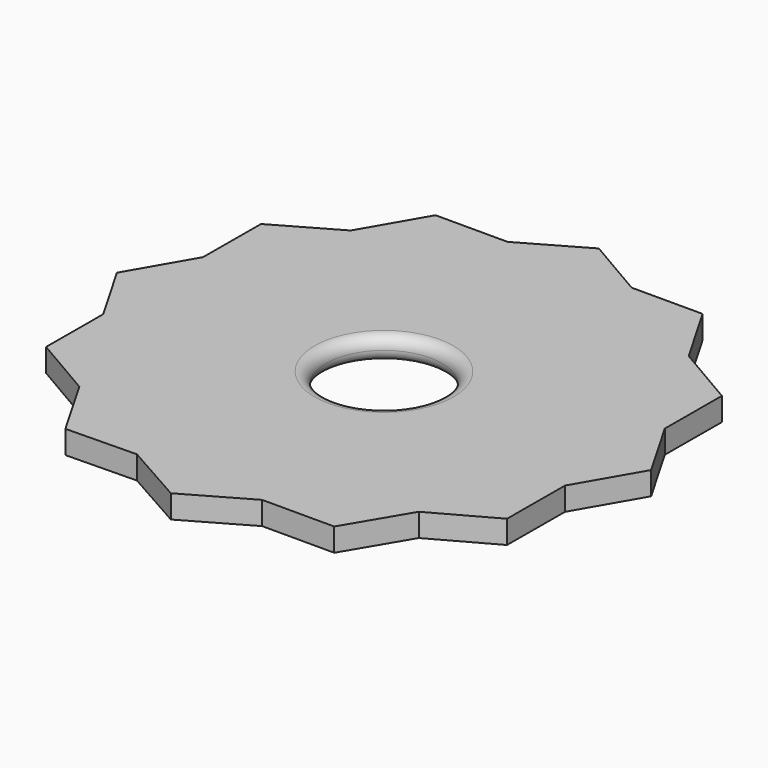
from build123d import *

# Parameters (mm, degrees)
F0_R     = 6.35
F1_DEPTH = 2.54
F2_R     = 1.26999


# Not quite as in the source:
# - a fillet or chamfer is up to 0.001 mm smaller than in the source, because OpenCascade refuses the exact size


with BuildPart() as f1:
    # F0 (on Top) → F1 (new body)
    with BuildSketch(Plane.XY):
        with BuildLine():
            Line((0.1342973504, 29.3290862039), (12.5991438484, 22.0549671115))
            ThreePointArc((12.5991438484, 22.0549671115), (12.7000000903, 21.997045204), (12.8005900541, 21.9386620893))
            Line((12.8005900541, 21.9386620893), (6.8682756911, 25.4))
            Line((6.8682756911, 25.4), (0.1342973504, 29.3290862039))
        make_face()
        with BuildLine():
            ThreePointArc((-12.5991438484, 22.0549671115), (0, 25.4), (12.5991438484, 22.0549671115))
            Line((12.5991438484, 22.0549671115), (0.1342973504, 29.3290862039))
            Line((0.1342973504, 29.3290862039), (-6.7436197563, 25.4))
            Line((-6.7436197563, 25.4), (-12.5991438484, 22.0549671115))
        make_face()
        Polygon((-18.5629074106, 18.6481012287), (-12.5991438484, 22.0549671115), (-6.7436197563, 25.4), (-14.6646968374, 25.4), align=None)
        with BuildLine():
            ThreePointArc((-25.3997337218, 0.1163050384), (-21.9386621638, 12.8005899263), (-12.5991438484, 22.0549671115))
            Line((-12.5991438484, 22.0549671115), (-18.5629074106, 18.6481012287))
            Line((-18.5629074106, 18.6481012287), (-25.3325850472, 14.780848019))
            Line((-25.3325850472, 14.780848019), (-25.3688551343, 6.8598539776))
            Line((-25.3688551343, 6.8598539776), (-25.3997337218, 0.1163050384))
        make_face()
        with BuildLine():
            Line((18.625235378, 18.5401460224), (12.8005900541, 21.9386620893))
            ThreePointArc((12.8005900541, 21.9386620893), (12.8993470878, 21.8807414113), (12.9978420445, 21.822376181))
            Line((12.9978420446, 21.822376181), (25.4668823975, 14.5482381848))
            Line((25.4668823975, 14.5482381848), (18.625235378, 18.5401460224))
        make_face()
        Polygon((6.8682756911, 25.4), (12.8005900541, 21.9386620893), (18.625235378, 18.5401460224), (14.6646968374, 25.4), align=None)
        with BuildLine():
            Line((25.4668823975, 14.5482381848), (12.9978420446, 21.822376181))
            ThreePointArc((12.9978420445, 21.822376181), (22.0828574683, 12.550195458), (25.4, 0))
            ThreePointArc((25.4, 0), (25.3999334305, -0.0581525957), (25.3997337225, -0.1163048866))
            Line((25.3997337225, -0.1163048866), (25.4002662804, 0))
            Line((25.4002662804, 0), (25.4311831017, 6.7518987713))
            Line((25.4311831017, 6.7518987713), (25.4668823975, 14.5482381848))
        make_face()
        Polygon((-25.4002662804, 0), (-25.3997337218, 0.1163050384), (-25.3688551343, 6.8598539776), (-29.3293936748, 0), (-25.4311831017, -6.7518987713), align=None)
        with BuildLine():
            ThreePointArc((-21.9970455091, -12.6999995618), (-24.5495027703, -6.5178151043), (-25.3997337218, 0.1163050384))
            Line((-25.3997337218, 0.1163050384), (-25.4002662804, 0))
            Line((-25.4002662804, 0), (-25.4311831017, -6.7518987713))
            Line((-25.4311831017, -6.7518987713), (-21.9970455091, -12.6999995618))
        make_face()
        with BuildLine():
            ThreePointArc((-12.800589874, -21.9386621944), (-18.0015854544, -17.9193448856), (-21.9970455091, -12.6999995618))
            Line((-21.9970455091, -12.6999995618), (-18.625235378, -18.5401460224))
            Line((-18.625235378, -18.5401460224), (-12.800589874, -21.9386621944))
        make_face()
        Polygon((-18.625235378, -18.5401460224), (-21.9970455091, -12.6999995618), (-25.4311831017, -6.7518987713), (-25.4668823975, -14.5482381848), align=None)
        with BuildLine():
            Line((25.3688551343, -6.8598539776), (25.3997337225, -0.1163048866))
            ThreePointArc((25.3997337225, -0.1163048866), (22.6367712709, -11.5211365077), (15.0421744156, -20.4668754052))
            Line((15.0421744156, -20.4668754052), (18.6118299226, -18.4944410973))
            Line((18.6118299226, -18.4944410973), (25.3325850472, -14.780848019))
            Line((25.3325850472, -14.780848019), (25.3688551343, -6.8598539776))
        make_face()
        Polygon((25.4002662804, 0), (25.3997337225, -0.1163048866), (25.3688551343, -6.8598539776), (29.3293936748, 0), (25.4311831017, 6.7518987713), align=None)
        with BuildLine():
            ThreePointArc((-12.1717221157, -22.2937027149), (-12.4874178664, -22.1184175526), (-12.800589874, -21.9386621944))
            Line((-12.800589874, -21.9386621944), (-18.625235378, -18.5401460224))
            Line((-18.625235378, -18.5401460224), (-14.6646968374, -25.4))
            Line((-14.6646968374, -25.4), (-6.9223574365, -25.2573419592))
            Line((-6.9223574365, -25.2573419592), (-12.1717221157, -22.2937027149))
        make_face()
        with BuildLine():
            Line((18.6118299226, -18.4944410973), (15.0421744156, -20.4668754052))
            ThreePointArc((15.0421744156, -20.4668754052), (12.4565037471, -22.1358423015), (9.6879678482, -23.4798483592))
            Line((9.6879678482, -23.4798483592), (6.7447131478, -25.1612151536))
            Line((6.7447131478, -25.1612151536), (14.6657902289, -25.1612151536))
            Line((14.6657902289, -25.1612151536), (18.6118299226, -18.4944410973))
        make_face()
        with BuildLine():
            ThreePointArc((9.6879678482, -23.4798483592), (-1.3762246139, -25.3626892465), (-12.1717221157, -22.2937027149))
            Line((-12.1717221157, -22.2937027149), (-6.9223574365, -25.2573419592))
            Line((-6.9223574365, -25.2573419592), (-0.1332039589, -29.0903013575))
            Line((-0.1332039589, -29.0903013575), (6.7447131478, -25.1612151536))
            Line((6.7447131478, -25.1612151536), (9.6879678482, -23.4798483592))
        make_face()
        with BuildLine():
            Line((12.9978420446, 21.822376181), (12.5991438484, 22.0549671115))
            ThreePointArc((12.5991438484, 22.0549671115), (0, 25.4), (-12.5991438484, 22.0549671115))
            ThreePointArc((-12.5991438484, 22.0549671115), (-21.9386621638, 12.8005899263), (-25.3997337218, 0.1163050384))
            ThreePointArc((-25.3997337218, 0.1163050384), (-24.5495027703, -6.5178151043), (-21.9970455091, -12.6999995618))
            ThreePointArc((-21.9970455091, -12.6999995618), (-18.0015854544, -17.9193448856), (-12.800589874, -21.9386621944))
            Line((-12.800589874, -21.9386621944), (-12.1717221157, -22.2937027149))
            ThreePointArc((-12.1717221157, -22.2937027149), (-1.3762246139, -25.3626892465), (9.6879678482, -23.4798483592))
            Line((9.6879678482, -23.4798483592), (12.6002372398, -21.8161822651))
            Line((12.6002372398, -21.8161822651), (15.0421744156, -20.4668754052))
            ThreePointArc((15.0421744156, -20.4668754052), (22.6367712709, -11.5211365077), (25.3997337225, -0.1163048866))
            ThreePointArc((25.3997337225, -0.1163048866), (25.3999334305, -0.0581525957), (25.4, 0))
            ThreePointArc((25.4, 0), (22.0828574683, 12.550195458), (12.9978420445, 21.822376181))
        make_face()
        Circle(F0_R, mode=Mode.SUBTRACT)
        with BuildLine():
            ThreePointArc((9.6879678482, -23.4798483592), (12.4565037471, -22.1358423015), (15.0421744156, -20.4668754052))
            Line((15.0421744156, -20.4668754052), (12.6002372398, -21.8161822651))
            Line((12.6002372398, -21.8161822651), (9.6879678482, -23.4798483592))
        make_face()
    extrude(amount=F1_DEPTH)

    # F2 (radius 1.27 in the source; OpenCascade refuses exactly that, so slightly less here)
    f2_edges = [f1.edges().sort_by_distance(p)[0] for p in [
        (-6.35, 0, 2.54),
        (-6.35, 0, 0),
    ]]
    fillet(f2_edges, radius=F2_R)


solid = f1.part
